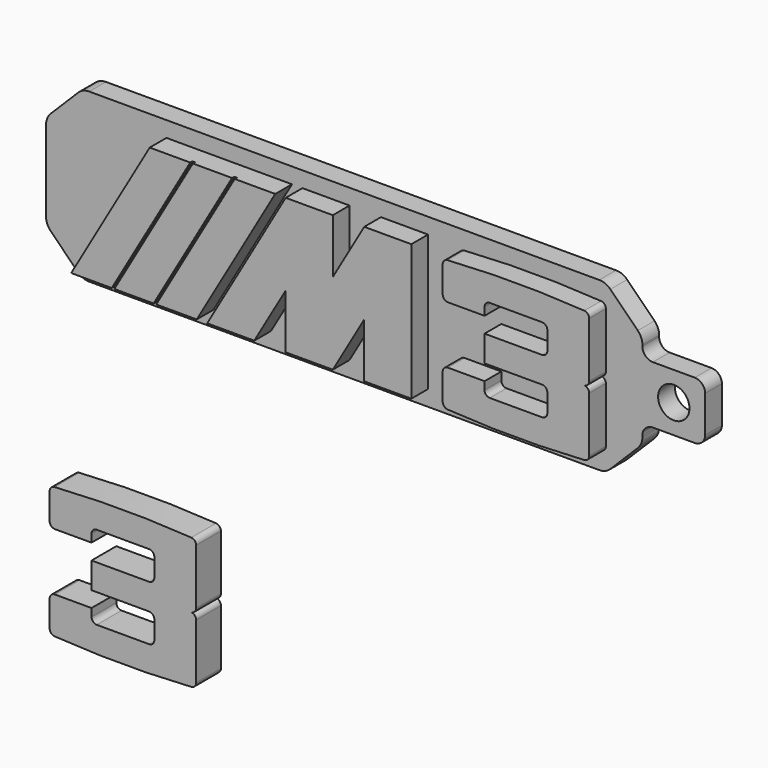
from build123d import *

# Parameters (mm, degrees)
F1_DEPTH  = 3.175
F3_DEPTH  = 3.175
F5_DEPTH  = 0.396875
F6_R      = 2.38125
F7_R      = 2.38125
F8_DEPTH  = 3.175
F11_DEPTH = 3.175
F12_DEPTH = 1.524


# Not quite as in the source:
# - a feature names something its author has since deleted; it is built from what else it names


with BuildPart() as f1:
    # F0 (on Front) → F1 (new body)
    with BuildSketch(Plane.XZ):
        Polygon((0, 5.55625), (5.55625, 0), (84.93125, 0), (90.4875, 5.55625), (90.4875, 19.84375), (84.93125, 25.4), (5.55625, 25.4), (0, 19.84375), align=None)
    extrude(amount=F1_DEPTH)

    # F2 (on face) → F3 (join)
    with BuildSketch(Plane.XZ.offset(3.175)):
        Polygon((18.2650661804, 23.01875), (6.35, 2.38125), (25.4, 2.38125), (37.3150661804, 23.01875), align=None)
        Polygon((38.9025661804, 23.01875), (26.9875, 2.38125), (34.13125, 2.38125), (38.9025661804, 10.6454120434), (38.9025661804, 2.38125), (46.0463161804, 2.38125), (50.8176323608, 10.6454120434), (50.8176323608, 2.38125), (57.9613823608, 2.38125), (57.9613823608, 23.01875), (50.8176323608, 23.01875), (46.0463161804, 14.7545879566), (46.0463161804, 23.01875), align=None)
        with BuildLine():
            ThreePointArc((63.4647834492, 22.6730891893), (62.9379825156, 22.4233597915), (62.7238823608, 21.8811005183))
            Line((62.7238823608, 21.8811005183), (62.7238823608, 17.859375))
            ThreePointArc((62.7238823608, 17.859375), (62.9563663532, 17.2981089924), (63.5176323608, 17.065625))
            Line((63.5176323608, 17.065625), (69.0738823608, 17.065625))
            Line((69.0738823608, 17.065625), (69.0738823608, 18.25625))
            ThreePointArc((69.0738823608, 18.25625), (69.3063663532, 18.8175160076), (69.8676323608, 19.05))
            Line((69.8676323608, 19.05), (77.8051323608, 19.05))
            ThreePointArc((77.8051323608, 19.05), (78.3663983684, 18.8175160076), (78.5988823608, 18.25625))
            Line((78.5988823608, 18.25625), (78.5988823608, 15.478125))
            ThreePointArc((78.5988823608, 15.478125), (78.3663983684, 14.9168589924), (77.8051323608, 14.684375))
            Line((77.8051323608, 14.684375), (69.0738823608, 14.684375))
            Line((69.0738823608, 14.684375), (69.0738823608, 10.715625))
            Line((69.0738823608, 10.715625), (77.8051323608, 10.715625))
            ThreePointArc((77.8051323608, 10.715625), (78.3663983684, 10.4831410076), (78.5988823608, 9.921875))
            Line((78.5988823608, 9.921875), (78.5988823608, 7.14375))
            ThreePointArc((78.5988823608, 7.14375), (78.3663983684, 6.5824839924), (77.8051323608, 6.35))
            Line((77.8051323608, 6.35), (69.8676323608, 6.35))
            ThreePointArc((69.8676323608, 6.35), (69.3063663532, 6.5824839924), (69.0738823608, 7.14375))
            Line((69.0738823608, 7.14375), (69.0738823608, 8.334375))
            Line((69.0738823608, 8.334375), (63.5176323608, 8.334375))
            ThreePointArc((63.5176323608, 8.334375), (62.9563663532, 8.1018910076), (62.7238823608, 7.540625))
            Line((62.7238823608, 7.540625), (62.7238823608, 3.5188994817))
            ThreePointArc((62.7238823608, 3.5188994817), (62.9379825156, 2.9766402085), (63.4647834492, 2.7269108107))
            ThreePointArc((63.4647834492, 2.7269108107), (73.8363823608, 2.38125), (84.2079812725, 2.7269108107))
            ThreePointArc((84.2079812725, 2.7269108107), (84.734782206, 2.9766402085), (84.9488823608, 3.5188994817))
            Line((84.9488823608, 3.5188994817), (84.9488823608, 11.90625))
            ThreePointArc((84.9488823608, 11.90625), (84.7163983684, 12.4675160076), (84.1551323608, 12.7))
            ThreePointArc((84.1551323608, 12.7), (84.7163983684, 12.9324839924), (84.9488823608, 13.49375))
            Line((84.9488823608, 13.49375), (84.9488823608, 16.8671875))
            Line((84.9488823608, 16.8671875), (84.9488823608, 21.8811005183))
            ThreePointArc((84.9488823608, 21.8811005183), (84.734782206, 22.4233597915), (84.2079812725, 22.6730891893))
            ThreePointArc((84.2079812725, 22.6730891893), (73.8363823608, 23.01875), (63.4647834492, 22.6730891893))
        make_face()
    extrude(amount=F3_DEPTH)

    # F4 (on face) → F5 (cut)
    with BuildSketch(Plane.XZ.offset(6.35)):
        Polygon((19.2484375, 2.38125), (31.1635036804, 23.01875), (30.7666286804, 23.01875), (18.8515625, 2.38125), align=None)
        Polygon((12.8984375, 2.38125), (24.8135036804, 23.01875), (24.4166286804, 23.01875), (12.5015625, 2.38125), align=None)
    extrude(amount=-F5_DEPTH, mode=Mode.SUBTRACT)

    # F6
    f6_edges = [f1.edges().sort_by_distance(p)[0] for p in [
        (90.4875, -1.5875, 19.84375),
        (84.93125, -1.5875, 25.4),
        (5.55625, -1.5875, 25.4),
        (5.55625, -1.5875, 0),
        (0, -1.5875, 5.55625),
        (0, -1.5875, 19.84375),
        (84.93125, -1.5875, 0),
        (90.4875, -1.5875, 5.55625),
    ]]
    fillet(f6_edges, radius=F6_R)

    # F7 (on face) → F8 (join, through all)
    with BuildSketch(Plane.XZ.offset(3.175)):
        with BuildLine():
            ThreePointArc((98.425, 8.334375), (99.5475320151, 8.7993429849), (100.0125, 9.921875))
            Line((100.0125, 9.921875), (100.0125, 15.478125))
            ThreePointArc((100.0125, 15.478125), (99.5475320151, 16.6006570151), (98.425, 17.065625))
            Line((98.425, 17.065625), (92.075, 17.065625))
            ThreePointArc((92.075, 17.065625), (90.9524679849, 17.5305929849), (90.4875, 18.653125))
            Line((90.4875, 18.653125), (90.4875, 6.746875))
            ThreePointArc((90.4875, 6.746875), (90.9524679849, 7.8694070151), (92.075, 8.334375))
            Line((92.075, 8.334375), (98.425, 8.334375))
        make_face()
        with Locations((95.25, 12.7)):
            Circle(F7_R, mode=Mode.SUBTRACT)
    extrude(amount=-F8_DEPTH)


with BuildPart() as f11:
    # F10 (on offset) → F11 (new body)
    with BuildSketch(Plane.XZ.offset(76.2)):
        with BuildLine():
            ThreePointArc((63.4647834492, 22.6730891893), (62.9379825156, 22.4233597915), (62.7238823608, 21.8811005183))
            Line((62.7238823608, 21.8811005183), (62.7238823608, 17.859375))
            ThreePointArc((62.7238823608, 17.859375), (62.9563663532, 17.2981089924), (63.5176323608, 17.065625))
            Line((63.5176323608, 17.065625), (69.0738823608, 17.065625))
            Line((69.0738823608, 17.065625), (69.0738823608, 18.25625))
            ThreePointArc((69.0738823608, 18.25625), (69.3063663532, 18.8175160076), (69.8676323608, 19.05))
            Line((69.8676323608, 19.05), (77.8051323608, 19.05))
            ThreePointArc((77.8051323608, 19.05), (78.3663983684, 18.8175160076), (78.5988823608, 18.25625))
            Line((78.5988823608, 18.25625), (78.5988823608, 15.478125))
            ThreePointArc((78.5988823608, 15.478125), (78.3663983684, 14.9168589924), (77.8051323608, 14.684375))
            Line((77.8051323608, 14.684375), (69.0738823608, 14.684375))
            Line((69.0738823608, 14.684375), (69.0738823608, 12.7))
            Line((69.0738823608, 12.7), (69.0738823608, 10.715625))
            Line((69.0738823608, 10.715625), (77.8051323608, 10.715625))
            ThreePointArc((77.8051323608, 10.715625), (78.3663983684, 10.4831410076), (78.5988823608, 9.921875))
            Line((78.5988823608, 9.921875), (78.5988823608, 7.14375))
            ThreePointArc((78.5988823608, 7.14375), (78.3663983684, 6.5824839924), (77.8051323608, 6.35))
            Line((77.8051323608, 6.35), (69.8676323608, 6.35))
            ThreePointArc((69.8676323608, 6.35), (69.3063663532, 6.5824839924), (69.0738823608, 7.14375))
            Line((69.0738823608, 7.14375), (69.0738823608, 8.334375))
            Line((69.0738823608, 8.334375), (63.5176323608, 8.334375))
            ThreePointArc((63.5176323608, 8.334375), (62.9563663532, 8.1018910076), (62.7238823608, 7.540625))
            Line((62.7238823608, 7.540625), (62.7238823608, 3.5188994817))
            ThreePointArc((62.7238823608, 3.5188994817), (62.9379825156, 2.9766402085), (63.4647834492, 2.7269108107))
            ThreePointArc((63.4647834492, 2.7269108107), (73.8363823608, 2.38125), (84.2079812725, 2.7269108107))
            ThreePointArc((84.2079812725, 2.7269108107), (84.734782206, 2.9766402085), (84.9488823608, 3.5188994817))
            Line((84.9488823608, 3.5188994817), (84.9488823608, 11.90625))
            ThreePointArc((84.9488823608, 11.90625), (84.7163983684, 12.4675160076), (84.1551323608, 12.7))
            ThreePointArc((84.1551323608, 12.7), (84.7163983684, 12.9324839924), (84.9488823608, 13.49375))
            Line((84.9488823608, 13.49375), (84.9488823608, 16.8671875))
            Line((84.9488823608, 16.8671875), (84.9488823608, 21.8811005183))
            ThreePointArc((84.9488823608, 21.8811005183), (84.734782206, 22.4233597915), (84.2079812725, 22.6730891893))
            ThreePointArc((84.2079812725, 22.6730891893), (73.8363823608, 23.01875), (63.4647834492, 22.6730891893))
        make_face()
    extrude(amount=F11_DEPTH)

    # F12 (add): a face of the model
    f12_faces = [f11.faces().sort_by_distance(p)[0] for p in [
        (75.2419009789, -79.375, 12.7),
    ]]
    extrude(f12_faces, amount=F12_DEPTH)


solid = Compound([f1.part, f11.part])
